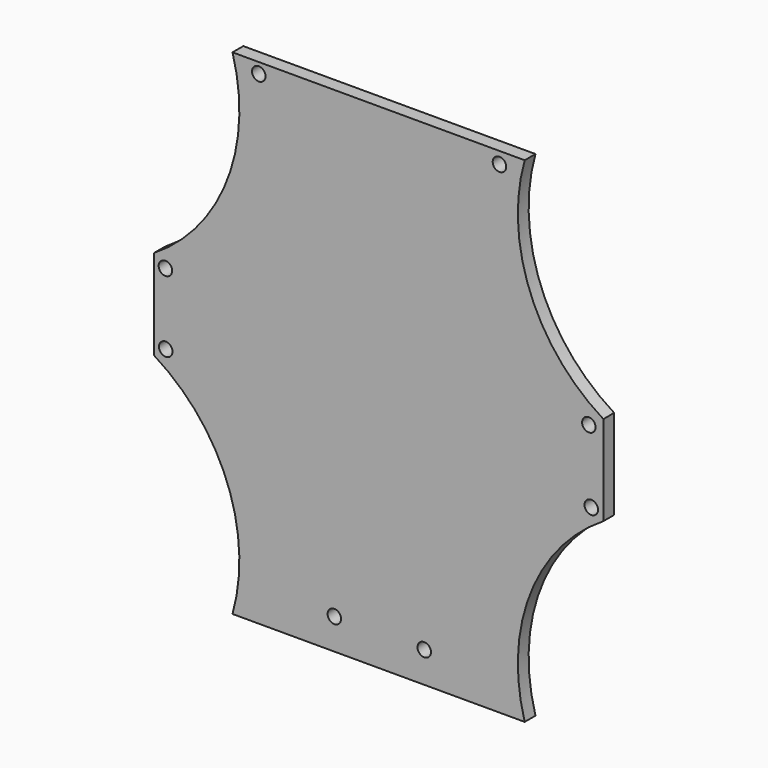
from build123d import *

# Parameters (mm, degrees)
F0_W      = 100
F0_H      = 110
F1_DEPTH  = 3
F3_DEPTH  = 25
F4_W      = 15
F4_H      = 6
F5_DEPTH  = 30
F6_R      = 3
F7_R      = 2.99999
F8_R      = 1.5
F9_DEPTH  = 25
F10_R     = 1.5
F11_DEPTH = 25
F12_R     = 1.5
F13_DEPTH = 25
F14_R     = 1.5
F15_DEPTH = 25


# Not quite as in the source:
# - a fillet or chamfer is up to 0.001 mm smaller than in the source, because OpenCascade refuses the exact size


with BuildPart() as f1:
    # F0 (on Front) → F1 (new body)
    with BuildSketch(Plane.XZ):
        with Locations((50, 55)):
            Rectangle(F0_W, F0_H)
    extrude(amount=F1_DEPTH)

    # F2 (on face) → F3 (cut)
    with BuildSketch(Plane.XZ.offset(3)):
        with BuildLine():
            Line((0, 110), (0, 65))
            ThreePointArc((0, 65), (16.3054104548, 84.5617848231), (17.5, 110))
            Line((17.5, 110), (0, 110))
        make_face()
        with BuildLine():
            Line((100, 110), (82.5, 110))
            ThreePointArc((82.5, 110), (83.6945895452, 84.5617848231), (100, 65))
            Line((100, 65), (100, 110))
        make_face()
        with BuildLine():
            ThreePointArc((100, 45), (83.6945895452, 25.4382151769), (82.5, 0))
            Line((82.5, 0), (100, 0))
            Line((100, 0), (100, 45))
        make_face()
        with BuildLine():
            Line((0, 45), (0, 0))
            Line((0, 0), (17.5, 0))
            ThreePointArc((17.5, 0), (16.3054104548, 25.4382151769), (0, 45))
        make_face()
    extrude(amount=-F3_DEPTH, mode=Mode.SUBTRACT)

    # F4 (on face) → F5 (join)
    with BuildSketch(Plane(origin=(0, 0, 0), x_dir=(-1, 0, 0), z_dir=(0, 1, 0))):
        with Locations((-50, 7)):
            Rectangle(F4_W, F4_H)
    extrude(amount=F5_DEPTH)

    # F6
    f6_edges = [f1.edges().sort_by_distance(p)[0] for p in [
        (50, 30, 4),
    ]]
    fillet(f6_edges, radius=F6_R)

    # F7 (radius 3 in the source; OpenCascade refuses exactly that, so slightly less here)
    f7_edges = [f1.edges().sort_by_distance(p)[0] for p in [
        (50, 30, 10),
    ]]
    fillet(f7_edges, radius=F7_R)

    # F8 (on face) → F9 (cut)
    with BuildSketch(Plane(origin=(0, 0, 0), x_dir=(-1, 0, 0), z_dir=(0, 1, 0))):
        with Locations((-40.1520836353, 6.8762069568)):
            Circle(F8_R)
        with Locations((-60.1520836353, 6.8762069568)):
            Circle(F8_R)
    extrude(amount=-F9_DEPTH, mode=Mode.SUBTRACT)

    # F10 (on face) → F11 (cut)
    with BuildSketch(Plane.XZ.offset(3)):
        with Locations((23.3403220773, 107.6833680272)):
            Circle(F10_R)
        with Locations((76.8845230341, 107.3717549443)):
            Circle(F10_R)
    extrude(amount=-F11_DEPTH, mode=Mode.SUBTRACT)

    # F12 (on face) → F13 (cut)
    with BuildSketch(Plane.XZ.offset(3)):
        with Locations((96.7704804272, 62.8292252972)):
            Circle(F12_R)
        with Locations((97.3125401127, 46.8384100805)):
            Circle(F12_R)
        with Locations((2.5671770603, 62.836966732)):
            Circle(F12_R)
    extrude(amount=-F13_DEPTH, mode=Mode.SUBTRACT)

    # F14 (on face) → F15 (cut)
    with BuildSketch(Plane.XZ.offset(3)):
        with Locations((2.6400329079, 47.0330864191)):
            Circle(F14_R)
    extrude(amount=-F15_DEPTH, mode=Mode.SUBTRACT)


solid = f1.part
